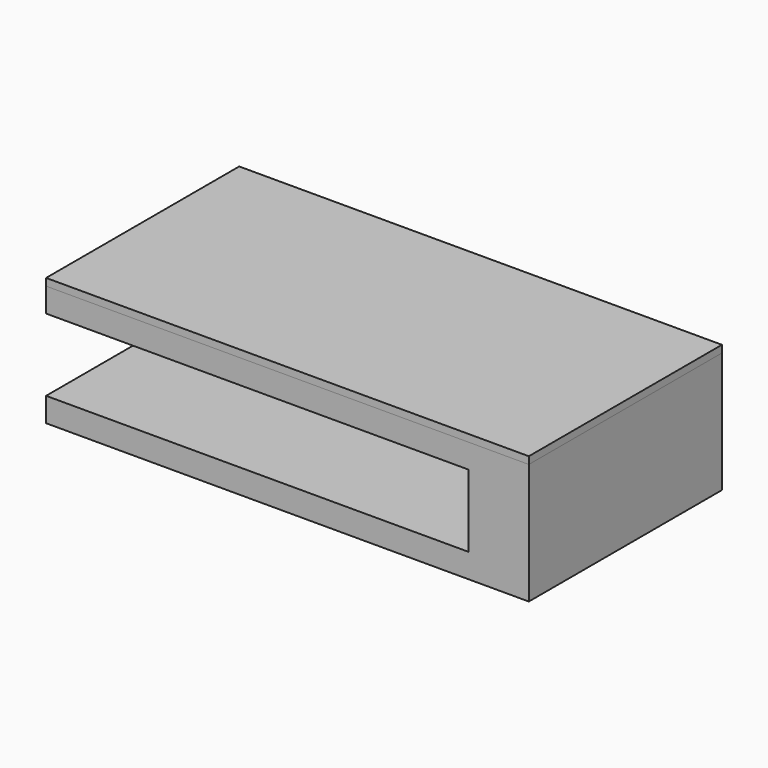
from build123d import *

# Parameters (mm, degrees)
F1_DEPTH = 1000
F3_W     = 2000
F3_H     = 30
F4_DEPTH = 1000


# Not quite as in the source:
# - a feature names something its author has since deleted; it is built from what else it names


with BuildPart() as f1:
    # F0 (on Front) → F1 (new body)
    with BuildSketch(Plane.XZ):
        Polygon((-2000, 0), (0, 0), (0, 500), (-2000, 500), (-2000, 400), (-250, 400), (-250, 100), (-2000, 100), align=None)
    extrude(amount=F1_DEPTH)


with BuildPart() as f4:
    # F3 (on face) → F4 (new body)
    with BuildSketch(Plane.XZ.offset(1000)):
        with Locations((-1000, 515)):
            Rectangle(F3_W, F3_H)
    extrude(amount=-F4_DEPTH)


solid = Compound([f1.part, f4.part])
